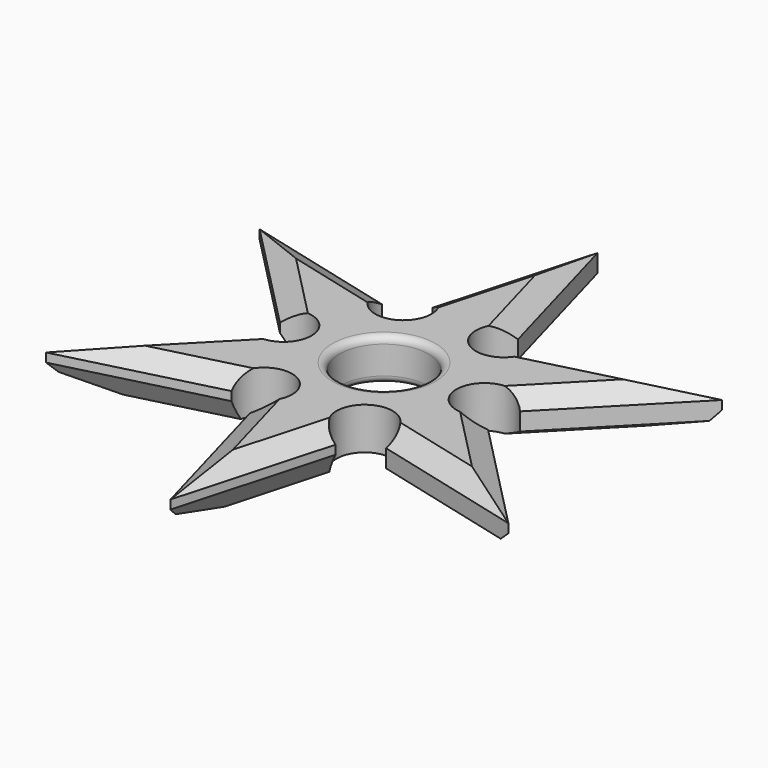
from build123d import *

# Parameters (mm, degrees)
F0_R         = 6.35
F1_DEPTH     = 6
F2_C1_SIZE2  = 3
F2_C1_SIZE   = 1.7320508076
F2_C2_SIZE2  = 3
F2_C2_SIZE   = 1.7320508076
F2_C3_SIZE2  = 3
F2_C3_SIZE   = 1.7320508076
F2_C4_SIZE2  = 3
F2_C4_SIZE   = 1.7320508076
F2_C5_SIZE2  = 1.7320508076
F2_C5_SIZE   = 3
F2_C6_SIZE2  = 3
F2_C6_SIZE   = 1.7320508076
F2_C7_SIZE2  = 3
F2_C7_SIZE   = 1.7320508076
F2_C8_SIZE2  = 3
F2_C8_SIZE   = 1.7320508076
F2_C9_SIZE2  = 1.7320508076
F2_C9_SIZE   = 3
F2_C10_SIZE2 = 3
F2_C10_SIZE  = 1.7320508076
F2_C11_SIZE2 = 1.7320508076
F2_C11_SIZE  = 3
F2_C12_SIZE2 = 3
F2_C12_SIZE  = 1.7320508076
F2_C13_SIZE2 = 1.7320508076
F2_C13_SIZE  = 3
F2_C14_SIZE2 = 3
F2_C14_SIZE  = 1.7320508076
F2_C15_SIZE2 = 3
F2_C15_SIZE  = 1.7320508076
F2_C16_SIZE2 = 3
F2_C16_SIZE  = 1.7320508076
F2_C17_SIZE2 = 1.7320508076
F2_C17_SIZE  = 3
F2_C18_SIZE2 = 3
F2_C18_SIZE  = 1.7320508076
F2_C19_SIZE2 = 3
F2_C19_SIZE  = 1.7320508076
F2_C20_SIZE2 = 3
F2_C20_SIZE  = 1.7320508076
F2_C21_SIZE2 = 1.7320508076
F2_C21_SIZE  = 3
F2_C22_SIZE2 = 3
F2_C22_SIZE  = 1.7320508076
F2_C23_SIZE2 = 3
F2_C23_SIZE  = 1.7320508076
F2_C24_SIZE2 = 3
F2_C24_SIZE  = 1.7320508076
F3_R         = 1


with BuildPart() as f1:
    # F0 (on Top) → F1 (new body)
    with BuildSketch(Plane.XY):
        with BuildLine():
            Line((6.0983324846, 16.2798387553), (0, 38.1))
            Line((0, 38.1), (-6.0983324846, 16.2798387553))
            ThreePointArc((-6.0983324846, 16.2798387553), (-5.175, 8.9633629292), (-11.0495876893, 13.42123023))
            Line((-11.0495876893, 13.42123023), (-32.9955678842, 19.05))
            Line((-32.9955678842, 19.05), (-17.1479201739, 2.8586085253))
            ThreePointArc((-17.1479201739, 2.8586085253), (-10.35, 0), (-17.1479201739, -2.8586085253))
            Line((-17.1479201739, -2.8586085253), (-32.9955678842, -19.05))
            Line((-32.9955678842, -19.05), (-11.0495876893, -13.42123023))
            ThreePointArc((-11.0495876893, -13.42123023), (-5.175, -8.9633629292), (-6.0983324846, -16.2798387553))
            Line((-6.0983324846, -16.2798387553), (0, -38.1))
            Line((0, -38.1), (6.0983324846, -16.2798387553))
            ThreePointArc((6.0983324846, -16.2798387553), (5.175, -8.9633629292), (11.0495876893, -13.42123023))
            Line((11.0495876893, -13.42123023), (32.9955678842, -19.05))
            Line((32.9955678842, -19.05), (17.1479201739, -2.8586085253))
            ThreePointArc((17.1479201739, -2.8586085253), (10.35, 0), (17.1479201739, 2.8586085253))
            Line((17.1479201739, 2.8586085253), (32.9955678842, 19.05))
            Line((32.9955678842, 19.05), (11.0495876893, 13.42123023))
            ThreePointArc((11.0495876893, 13.42123023), (5.175, 8.9633629292), (6.0983324846, 16.2798387553))
        make_face()
        Circle(F0_R, mode=Mode.SUBTRACT)
    extrude(amount=F1_DEPTH)

    # F2: chamfer of 3 x 1.7320508076 on 24 edges, made by hand

    # F2_c1
    f2_c1_edges = [f1.edges().sort_by_distance(p)[0] for p in [
        (22.0225777867, -16.235615115, 0),
    ]]
    f2_c1_side = f1.faces().sort_by_distance((22.0225777867, -16.235615115, 0.0346410162))[0]
    chamfer(f2_c1_edges, length=F2_C1_SIZE, length2=F2_C1_SIZE2, reference=f2_c1_side)

    # F2_c2
    f2_c2_edges = [f1.edges().sort_by_distance(p)[0] for p in [
        (22.0225777867, -16.235615115, 6),
    ]]
    f2_c2_side = f1.faces().sort_by_distance((22.0225777867, -16.235615115, 5.9653589838))[0]
    chamfer(f2_c2_edges, length=F2_C2_SIZE, length2=F2_C2_SIZE2, reference=f2_c2_side)

    # F2_c3
    f2_c3_edges = [f1.edges().sort_by_distance(p)[0] for p in [
        (23.0480423242, -8.8867074098, 0),
    ]]
    f2_c3_side = f1.faces().sort_by_distance((23.0232860482, -8.9109381093, 0))[0]
    chamfer(f2_c3_edges, length=F2_C3_SIZE, length2=F2_C3_SIZE2, reference=f2_c3_side)

    # F2_c4
    f2_c4_edges = [f1.edges().sort_by_distance(p)[0] for p in [
        (23.0480423242, -8.8867074098, 6),
    ]]
    f2_c4_side = f1.faces().sort_by_distance((23.0480423242, -8.8867074098, 5.9653589838))[0]
    chamfer(f2_c4_edges, length=F2_C4_SIZE, length2=F2_C4_SIZE2, reference=f2_c4_side)

    # F2_c5
    f2_c5_edges = [f1.edges().sort_by_distance(p)[0] for p in [
        (25.071744029, 10.9543042626, 0),
    ]]
    f2_c5_side = f1.faces().sort_by_distance((25.046987753, 10.9785349621, 0))[0]
    chamfer(f2_c5_edges, length=F2_C5_SIZE, length2=F2_C5_SIZE2, reference=f2_c5_side)

    # F2_c6
    f2_c6_edges = [f1.edges().sort_by_distance(p)[0] for p in [
        (25.071744029, 10.9543042626, 6),
    ]]
    f2_c6_side = f1.faces().sort_by_distance((25.071744029, 10.9543042626, 5.9653589838))[0]
    chamfer(f2_c6_edges, length=F2_C6_SIZE, length2=F2_C6_SIZE2, reference=f2_c6_side)

    # F2_c7
    f2_c7_edges = [f1.edges().sort_by_distance(p)[0] for p in [
        (19.220135535, 15.5168364554, 0),
    ]]
    f2_c7_side = f1.faces().sort_by_distance((19.2287417983, 15.4832815417, 0))[0]
    chamfer(f2_c7_edges, length=F2_C7_SIZE, length2=F2_C7_SIZE2, reference=f2_c7_side)

    # F2_c8
    f2_c8_edges = [f1.edges().sort_by_distance(p)[0] for p in [
        (19.220135535, 15.5168364554, 6),
    ]]
    f2_c8_side = f1.faces().sort_by_distance((19.220135535, 15.5168364554, 5.9653589838))[0]
    chamfer(f2_c8_edges, length=F2_C8_SIZE, length2=F2_C8_SIZE2, reference=f2_c8_side)

    # F2_c9
    f2_c9_edges = [f1.edges().sort_by_distance(p)[0] for p in [
        (3.0491662423, 27.1899193776, 0),
    ]]
    f2_c9_side = f1.faces().sort_by_distance((3.015803703, 27.1805951634, 0))[0]
    chamfer(f2_c9_edges, length=F2_C9_SIZE, length2=F2_C9_SIZE2, reference=f2_c9_side)

    # F2_c10
    f2_c10_edges = [f1.edges().sort_by_distance(p)[0] for p in [
        (3.0491662423, 27.1899193776, 6),
    ]]
    f2_c10_side = f1.faces().sort_by_distance((3.0491662423, 27.1899193776, 5.9653589838))[0]
    chamfer(f2_c10_edges, length=F2_C10_SIZE, length2=F2_C10_SIZE2, reference=f2_c10_side)

    # F2_c11
    f2_c11_edges = [f1.edges().sort_by_distance(p)[0] for p in [
        (-3.8279067892, 24.4035438652, 0),
    ]]
    f2_c11_side = f1.faces().sort_by_distance((-3.7945442499, 24.394219651, 0))[0]
    chamfer(f2_c11_edges, length=F2_C11_SIZE, length2=F2_C11_SIZE2, reference=f2_c11_side)

    # F2_c12
    f2_c12_edges = [f1.edges().sort_by_distance(p)[0] for p in [
        (-3.8279067892, 24.4035438652, 6),
    ]]
    f2_c12_side = f1.faces().sort_by_distance((-3.8279067892, 24.4035438652, 5.9653589838))[0]
    chamfer(f2_c12_edges, length=F2_C12_SIZE, length2=F2_C12_SIZE2, reference=f2_c12_side)

    # F2_c13
    f2_c13_edges = [f1.edges().sort_by_distance(p)[0] for p in [
        (-22.0225777867, 16.235615115, 0),
    ]]
    f2_c13_side = f1.faces().sort_by_distance((-22.03118405, 16.2020602013, 0))[0]
    chamfer(f2_c13_edges, length=F2_C13_SIZE, length2=F2_C13_SIZE2, reference=f2_c13_side)

    # F2_c14
    f2_c14_edges = [f1.edges().sort_by_distance(p)[0] for p in [
        (-22.0225777867, 16.235615115, 6),
    ]]
    f2_c14_side = f1.faces().sort_by_distance((-22.0225777867, 16.235615115, 5.9653589838))[0]
    chamfer(f2_c14_edges, length=F2_C14_SIZE, length2=F2_C14_SIZE2, reference=f2_c14_side)

    # F2_c15
    f2_c15_edges = [f1.edges().sort_by_distance(p)[0] for p in [
        (-23.0480423242, 8.8867074098, 0),
    ]]
    f2_c15_side = f1.faces().sort_by_distance((-23.0232860482, 8.9109381093, 0))[0]
    chamfer(f2_c15_edges, length=F2_C15_SIZE, length2=F2_C15_SIZE2, reference=f2_c15_side)

    # F2_c16
    f2_c16_edges = [f1.edges().sort_by_distance(p)[0] for p in [
        (-23.0480423242, 8.8867074098, 6),
    ]]
    f2_c16_side = f1.faces().sort_by_distance((-23.0480423242, 8.8867074098, 5.9653589838))[0]
    chamfer(f2_c16_edges, length=F2_C16_SIZE, length2=F2_C16_SIZE2, reference=f2_c16_side)

    # F2_c17
    f2_c17_edges = [f1.edges().sort_by_distance(p)[0] for p in [
        (-25.071744029, -10.9543042626, 0),
    ]]
    f2_c17_side = f1.faces().sort_by_distance((-25.046987753, -10.9785349621, 0))[0]
    chamfer(f2_c17_edges, length=F2_C17_SIZE, length2=F2_C17_SIZE2, reference=f2_c17_side)

    # F2_c18
    f2_c18_edges = [f1.edges().sort_by_distance(p)[0] for p in [
        (-25.071744029, -10.9543042626, 6),
    ]]
    f2_c18_side = f1.faces().sort_by_distance((-25.071744029, -10.9543042626, 5.9653589838))[0]
    chamfer(f2_c18_edges, length=F2_C18_SIZE, length2=F2_C18_SIZE2, reference=f2_c18_side)

    # F2_c19
    f2_c19_edges = [f1.edges().sort_by_distance(p)[0] for p in [
        (-19.220135535, -15.5168364554, 0),
    ]]
    f2_c19_side = f1.faces().sort_by_distance((-19.2287417983, -15.4832815417, 0))[0]
    chamfer(f2_c19_edges, length=F2_C19_SIZE, length2=F2_C19_SIZE2, reference=f2_c19_side)

    # F2_c20
    f2_c20_edges = [f1.edges().sort_by_distance(p)[0] for p in [
        (-19.220135535, -15.5168364554, 6),
    ]]
    f2_c20_side = f1.faces().sort_by_distance((-19.220135535, -15.5168364554, 5.9653589838))[0]
    chamfer(f2_c20_edges, length=F2_C20_SIZE, length2=F2_C20_SIZE2, reference=f2_c20_side)

    # F2_c21
    f2_c21_edges = [f1.edges().sort_by_distance(p)[0] for p in [
        (-3.0491662423, -27.1899193776, 0),
    ]]
    f2_c21_side = f1.faces().sort_by_distance((-3.015803703, -27.1805951634, 0))[0]
    chamfer(f2_c21_edges, length=F2_C21_SIZE, length2=F2_C21_SIZE2, reference=f2_c21_side)

    # F2_c22
    f2_c22_edges = [f1.edges().sort_by_distance(p)[0] for p in [
        (-3.0491662423, -27.1899193776, 6),
    ]]
    f2_c22_side = f1.faces().sort_by_distance((-3.0491662423, -27.1899193776, 5.9653589838))[0]
    chamfer(f2_c22_edges, length=F2_C22_SIZE, length2=F2_C22_SIZE2, reference=f2_c22_side)

    # F2_c23
    f2_c23_edges = [f1.edges().sort_by_distance(p)[0] for p in [
        (3.8279067892, -24.4035438652, 0),
    ]]
    f2_c23_side = f1.faces().sort_by_distance((3.7945442499, -24.394219651, 0))[0]
    chamfer(f2_c23_edges, length=F2_C23_SIZE, length2=F2_C23_SIZE2, reference=f2_c23_side)

    # F2_c24
    f2_c24_edges = [f1.edges().sort_by_distance(p)[0] for p in [
        (3.8279067892, -24.4035438652, 6),
    ]]
    f2_c24_side = f1.faces().sort_by_distance((3.8279067892, -24.4035438652, 5.9653589838))[0]
    chamfer(f2_c24_edges, length=F2_C24_SIZE, length2=F2_C24_SIZE2, reference=f2_c24_side)

    # F3
    f3_edges = [f1.edges().sort_by_distance(p)[0] for p in [
        (-6.35, 0, 0),
        (-6.35, 0, 6),
    ]]
    fillet(f3_edges, radius=F3_R)


solid = f1.part
